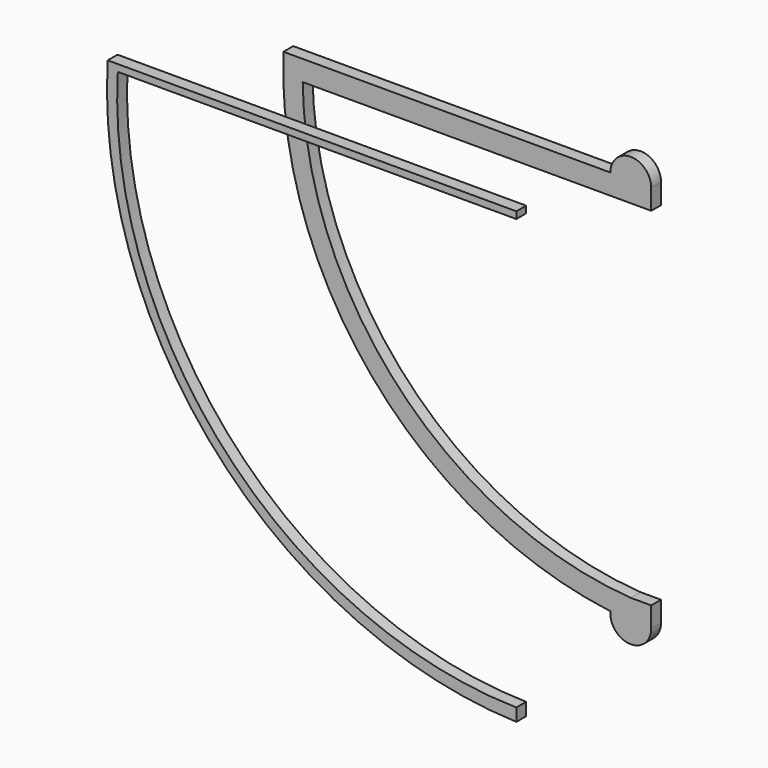
from build123d import *

# Parameters (mm, degrees)
F3_DEPTH = 3
F4_DEPTH = 3


# Not quite as in the source:
# - the program builds the solid bodies; features that only make, move or delete a surface that nothing else refers to are left out


with BuildPart() as f3:
    # F2 (on offset) → F3 (new body)
    with BuildSketch(Plane.XZ.offset(35)):
        with BuildLine():
            Line((0, 53.3243566751), (0, 55))
            Line((0, 55), (-100, 55))
            ThreePointArc((-100, 55), (-73.1778339448, -21.0707581316), (0, -55))
            Line((0, -55), (0, -51.8885441124))
            ThreePointArc((0, -51.8885441124), (-71.111364106, -19.9961360664), (-97.532135104, 53.3243566751))
            Line((-97.532135104, 53.3243566751), (0, 53.3243566751))
        make_face()
    extrude(amount=F3_DEPTH)


with BuildPart() as f4:
    # F0 (on Front) → F4 (new body)
    with BuildSketch(Plane.XZ):
        with BuildLine():
            Line((-5, 47.5), (0, 47.5))
            Line((0, 47.5), (5, 47.5))
            ThreePointArc((5, 47.5), (0, 52.5), (-5, 47.5))
        make_face()
        with BuildLine():
            Line((0, 42.5), (0, 47.5))
            Line((0, 47.5), (-5, 47.5))
            ThreePointArc((-5, 47.5), (-3.5355339059, 43.9644660941), (0, 42.5))
        make_face()
        with BuildLine():
            Line((5, 47.5), (0, 47.5))
            Line((0, 47.5), (0, 42.5))
            ThreePointArc((0, 42.5), (3.5355339059, 43.9644660941), (5, 47.5))
        make_face()
        with BuildLine():
            Line((-80.2852206571, 42.5), (0, 42.5))
            ThreePointArc((0, 42.5), (-3.5355339059, 43.9644660941), (-5, 47.5))
            Line((-5, 47.5), (-85, 47.5))
            ThreePointArc((-85, 47.5), (-63.3965803265, -15.3423221911), (-4.9760293042, -47.0109883803))
            ThreePointArc((-4.9760293042, -47.0109883803), (-3.3581945969, -43.7956067907), (0, -42.5))
            ThreePointArc((0, -42.5), (-56.7498093098, -15.6860309965), (-80.2852206571, 42.5))
        make_face()
        with BuildLine():
            ThreePointArc((5, -47.5), (3.5355339059, -43.9644660941), (0, -42.5))
            ThreePointArc((0, -42.5), (-3.3581945969, -43.7956067907), (-4.9760293042, -47.0109883803))
            ThreePointArc((-4.9760293042, -47.0109883803), (-2.4913542209, -47.289476598), (0, -47.5))
            Line((0, -47.5), (5, -47.5))
        make_face()
        with BuildLine():
            ThreePointArc((-4.9760293042, -47.0109883803), (-0.2447993865, -52.4940037305), (5, -47.5))
            Line((5, -47.5), (0, -47.5))
            ThreePointArc((0, -47.5), (-2.4913542209, -47.289476598), (-4.9760293042, -47.0109883803))
        make_face()
        with BuildLine():
            Line((5, -42.5), (0, -42.5))
            ThreePointArc((0, -42.5), (3.5355339059, -43.9644660941), (5, -47.5))
            Line((5, -47.5), (5, -42.5))
        make_face()
        with BuildLine():
            ThreePointArc((5, 47.5), (3.5355339059, 43.9644660941), (0, 42.5))
            Line((0, 42.5), (5, 42.5))
            Line((5, 42.5), (5, 47.5))
        make_face()
    extrude(amount=F4_DEPTH)


solid = Compound([f3.part, f4.part])
